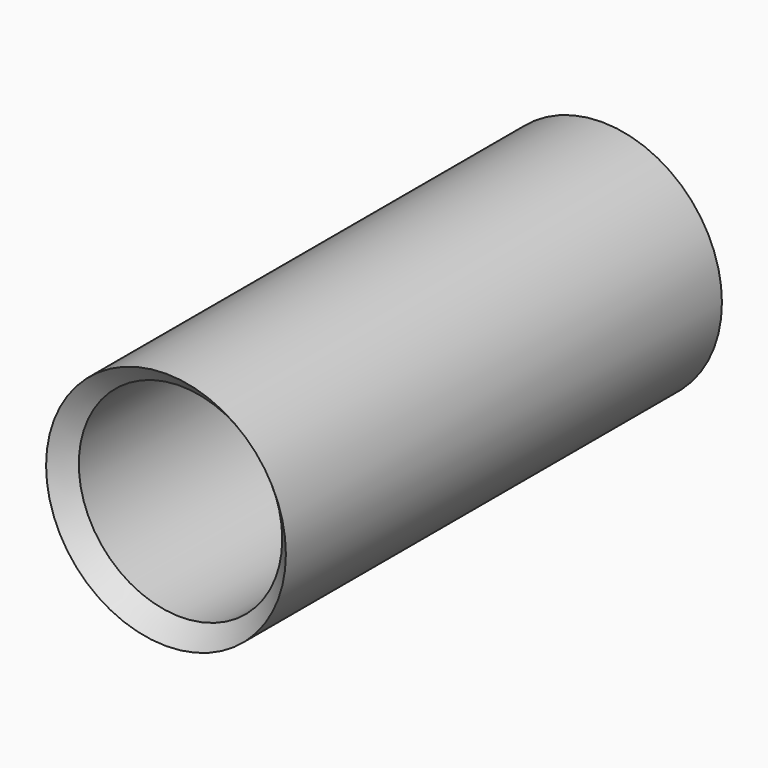
from build123d import *

# Parameters (mm, degrees)
F0_R     = 16.5
F0_R_2   = 14
F1_DEPTH = 38


# Not quite as in the source:
# - a fillet or chamfer that OpenCascade refuses, or shapes differently, is made with other operations: its cross-section is extruded or revolved along the edge and cut away or added


with BuildPart() as f1:
    # F0 (on Front) → F1 (new body, symmetric)
    with BuildSketch(Plane.XZ):
        Circle(F0_R)
        Circle(F0_R_2, mode=Mode.SUBTRACT)
    extrude(amount=F1_DEPTH, both=True)

    # F2: chamfer of 3 on 2 edges, made by hand

    # F2_s1 → F2_t2 (revolve, cut)
    with BuildSketch(Plane.XY):
        Polygon((17, -38), (14, -35), (14, -38), align=None)
    revolve(axis=Axis((0, -38, 0), (0, -1, 0)), mode=Mode.SUBTRACT)

    # F2_s3 → F2_t4 (revolve, cut)
    with BuildSketch(Plane.XY):
        Polygon((14, 35), (17, 38), (14, 38), align=None)
    revolve(axis=Axis((0, 38, 0), (0, -1, 0)), mode=Mode.SUBTRACT)


solid = f1.part
